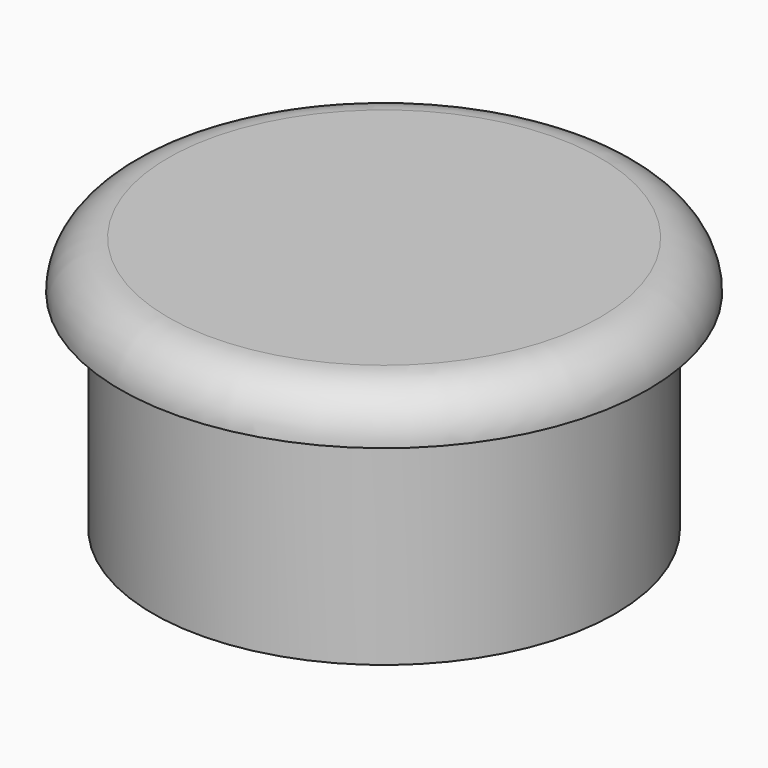
from build123d import *

# Parameters (mm, degrees)
F0_R     = 14.445
F0_R_2   = 12.945
F1_DEPTH = 13
F2_R     = 16.5
F3_DEPTH = 3
F4_R     = 2.99999


# Not quite as in the source:
# - a fillet or chamfer is up to 0.001 mm smaller than in the source, because OpenCascade refuses the exact size


with BuildPart() as f1:
    # F0 (on Top) → F1 (new body)
    with BuildSketch(Plane.XY):
        Circle(F0_R)
        Circle(F0_R_2, mode=Mode.SUBTRACT)
    extrude(amount=F1_DEPTH)

    # F2 (on face) → F3 (join)
    with BuildSketch(Plane.XY.offset(13)):
        Circle(F2_R)
    extrude(amount=F3_DEPTH)

    # F4 (radius 3 in the source; OpenCascade refuses exactly that, so slightly less here)
    f4_edges = [f1.edges().sort_by_distance(p)[0] for p in [
        (-16.5, 0, 16),
        (-12.945, 0, 13),
    ]]
    fillet(f4_edges, radius=F4_R)


solid = f1.part
